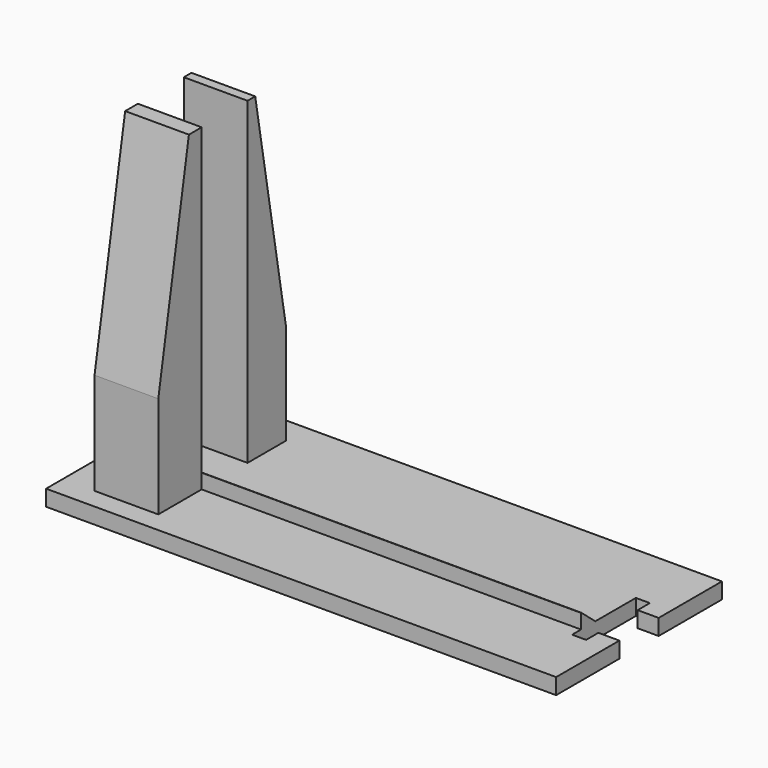
from build123d import *

# Parameters (mm, degrees)
F0_W     = 203.2
F0_H     = 82.55
F1_DEPTH = 6.35
F3_DEPTH = 25.4
F4_W     = 25.4
F4_H     = 21.59
F5_DEPTH = 127
F4_H_2   = 19.05
F6_SIZE2 = 15.24
F6_SIZE  = 86.430334931
F7_SIZE2 = 15.24
F7_SIZE  = 86.430334931
F4_W_2   = 151.13
F4_H_3   = 7.112
F8_DEPTH = 5.842
F9_SIZE2 = 6.962214
F9_SIZE  = 5.84199


# Not quite as in the source:
# - a fillet or chamfer is up to 0.001 mm smaller than in the source, because OpenCascade refuses the exact size
# - a feature names something its author has since deleted; it is built from what else it names


with BuildPart() as f1:
    # F0 (on Top) → F1 (new body)
    with BuildSketch(Plane.XY):
        with Locations((38.0131614566, -92.994289273)):
            Rectangle(F0_W, F0_H)
    extrude(amount=F1_DEPTH)

    # F2 (on face) → F3 (cut)
    with BuildSketch(Plane.XY.offset(6.35)):
        Polygon((131.2311614566, -83.215289273), (131.2311614566, -77.119289273), (125.6431614566, -77.119289273), (125.6431614566, -108.869289273), (131.2311614566, -108.869289273), (131.2311614566, -102.773289273), (139.6131614566, -102.773289273), (139.6131614566, -83.215289273), align=None)
    extrude(amount=-F3_DEPTH, mode=Mode.SUBTRACT)

    # F4 (on face) → F8 (join)
    with BuildSketch(Plane.XY.offset(6.35)):
        with Locations((50.0781614566, -100.868289273)):
            Rectangle(F4_W_2, F4_H_3)
        with Locations((-38.1868385434, -100.868289273)):
            Rectangle(F4_W, F4_H_3)
    extrude(amount=F8_DEPTH)

    # F9 (size 5.842 and 6.9622244879 in the source; OpenCascade refuses exactly that, so slightly less here)
    f9_edges = [f1.edges().sort_by_distance(p)[0] for p in [
        (37.378161, -97.312289, 12.192),
    ]]
    f9_side = f1.faces().sort_by_distance((37.378161, -97.312289, 9.271))[0]
    chamfer(f9_edges, length=F9_SIZE, length2=F9_SIZE2, reference=f9_side)


with BuildPart() as f5:
    # F4 (on face) → F5 (new body)
    with BuildSketch(Plane.XY.offset(6.35)):
        with Locations((-38.1868385434, -115.219289273)):
            Rectangle(F4_W, F4_H)
    extrude(amount=F5_DEPTH)

    # F6
    f6_edges = [f5.edges().sort_by_distance(p)[0] for p in [
        (-38.186839, -126.014289, 133.35),
    ]]
    f6_side = f5.faces().sort_by_distance((-38.186839, -126.014289, 69.85))[0]
    chamfer(f6_edges, length=F6_SIZE, length2=F6_SIZE2, reference=f6_side)


with BuildPart() as f5b:
    # F4 (on face) → F5, piece 2 (new body)
    with BuildSketch(Plane.XY.offset(6.35)):
        with Locations((-38.1868385434, -72.039289273)):
            Rectangle(F4_W, F4_H_2)
    extrude(amount=F5_DEPTH)

    # F7
    f7_edges = [f5b.edges().sort_by_distance(p)[0] for p in [
        (-38.186839, -62.514289, 133.35),
    ]]
    f7_side = f5b.faces().sort_by_distance((-38.186839, -62.514289, 69.85))[0]
    chamfer(f7_edges, length=F7_SIZE, length2=F7_SIZE2, reference=f7_side)


solid = Compound([f1.part, f5.part, f5b.part])
